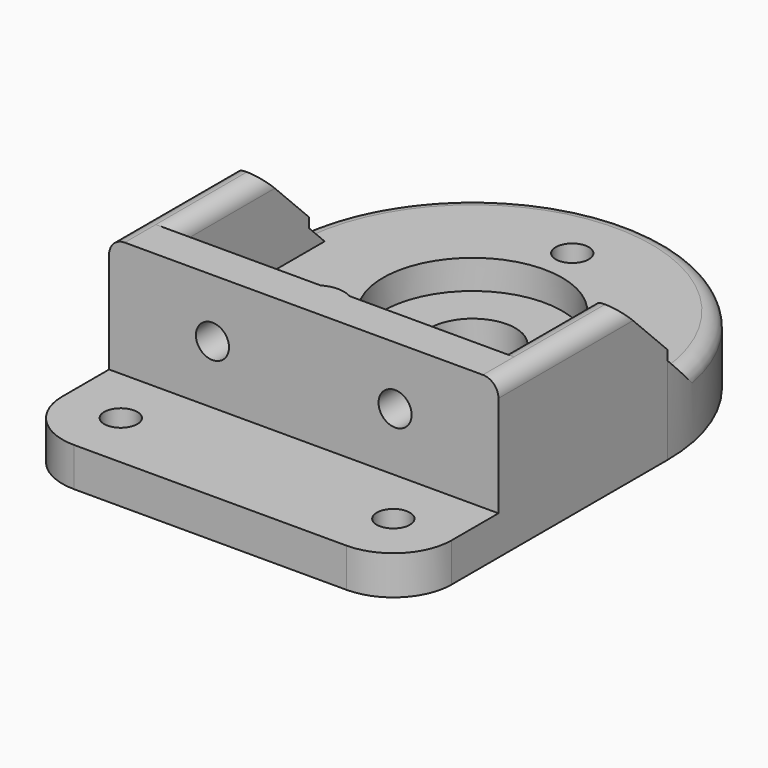
from build123d import *

# Parameters (mm, degrees)
F0_R          = 2.125
F0_R_2        = 5.25
F1_DEPTH      = 5
F3_DEPTH      = 15
F4_R          = 2.125
F5_DEPTH      = 25
F6_W          = 50
F6_H          = 15
F6_R          = 2.125
F7_DEPTH      = 5
F8_R          = 7.5
F9_SIZE       = 7.5
F10_R         = 2.125
F10_R_2       = 11.5
F11_DEPTH     = 3.75
F12_T1_DEPTH  = 10
F12_T6_DEPTH  = 4
F12_S7_R      = 25
F12_T8_DEPTH  = 4
F12_T12_DEPTH = 4
F12_S13_R     = 25
F12_T14_DEPTH = 4
F13_R         = 4.99999
F14_R         = 1.99999
F15_R         = 5.5
F16_DEPTH     = 25


# Not quite as in the source:
# - a fillet or chamfer that OpenCascade refuses, or shapes differently, is made with other operations: its cross-section is extruded or revolved along the edge and cut away or added
# - a fillet or chamfer is up to 0.001 mm smaller than in the source, because OpenCascade refuses the exact size


with BuildPart() as f1:
    # F0 (on Top) → F1 (new body)
    with BuildSketch(Plane.XY):
        with BuildLine():
            Line((25, -27.1), (25, -22.1))
            Line((25, -22.1), (25, 0))
            ThreePointArc((25, 0), (0, 25), (-25, 0))
            Line((-25, 0), (-25, -22.1))
            Line((-25, -22.1), (-25, -27.1))
            Line((-25, -27.1), (25, -27.1))
        make_face()
        with Locations((-13.8564064606, -8)):
            Circle(F0_R, mode=Mode.SUBTRACT)
        with Locations((13.8564064606, -8)):
            Circle(F0_R, mode=Mode.SUBTRACT)
        Circle(F0_R_2, mode=Mode.SUBTRACT)
        with Locations((0, 16)):
            Circle(F0_R, mode=Mode.SUBTRACT)
    extrude(amount=F1_DEPTH)

    # F2 (on face) → F3 (join)
    with BuildSketch(Plane.XY.offset(5)):
        Polygon((-25, -27.1), (25, -27.1), (25, -22.1), (25, 0), (21, 0), (21, -22.1), (5, -22.1), (5, -14.1), (0, -14.1), (-5, -14.1), (-5, -22.1), (-21, -22.1), (-21, 0), (-25, 0), (-25, -22.1), align=None)
    extrude(amount=F3_DEPTH)

    # F4 (on face) → F5 (cut)
    with BuildSketch(Plane.XZ.offset(27.1)):
        with Locations((-11.725, 12.5)):
            Circle(F4_R)
        with Locations((11.725, 12.5)):
            Circle(F4_R)
    extrude(amount=-F5_DEPTH, mode=Mode.SUBTRACT)

    # F6 (on Top) → F7 (join)
    with BuildSketch(Plane.XY):
        with Locations((0, -34.6)):
            Rectangle(F6_W, F6_H)
        with Locations((-17.5, -34.6)):
            Circle(F6_R, mode=Mode.SUBTRACT)
        with Locations((17.5, -34.6)):
            Circle(F6_R, mode=Mode.SUBTRACT)
    extrude(amount=F7_DEPTH)

    # F8
    f8_edges = [f1.edges().sort_by_distance(p)[0] for p in [
        (-25, -42.1, 2.5),
        (25, -42.1, 2.5),
    ]]
    fillet(f8_edges, radius=F8_R)

    # F9
    f9_edges = [f1.edges().sort_by_distance(p)[0] for p in [
        (0, -14.1, 20),
        (-23, 0, 20),
        (23, 0, 20),
    ]]
    chamfer(f9_edges, length=F9_SIZE)

    # F10 (on face) → F11 (join)
    with BuildSketch(Plane.XY.offset(5)):
        with BuildLine():
            Line((25, -22.1), (25, 0))
            ThreePointArc((25, 0), (0, 25), (-25, 0))
            Line((-25, 0), (-25, -22.1))
            Line((-25, -22.1), (25, -22.1))
        make_face()
        with Locations((-13.8564064606, -8)):
            Circle(F10_R, mode=Mode.SUBTRACT)
        Circle(F10_R_2, mode=Mode.SUBTRACT)
        with Locations((13.8564064606, -8)):
            Circle(F10_R, mode=Mode.SUBTRACT)
        with Locations((0, 16)):
            Circle(F10_R, mode=Mode.SUBTRACT)
    extrude(amount=F11_DEPTH)

    # F12: chamfer of 2.5 on 3 edges, made by hand

    # F12_s2 → F12_t1 (join)
    with BuildSketch(Plane.YZ.offset(-5)):
        with BuildLine():
            Line((-14.1707106781, 11.3207106781), (-11.5292893219, 8.6792893219))
            Line((-11.5292893219, 8.6792893219), (-11.5292893219, 8.6292893219))
            ThreePointArc((-11.5292893219, 8.6292893219), (-12.8146446609, 8.7), (-14.1, 8.7))
            Line((-14.1, 8.7), (-14.15, 8.75))
            ThreePointArc((-14.15, 8.75), (-14.15, 10.0353553391), (-14.2207106781, 11.3207106781))
            Line((-14.2207106781, 11.3207106781), (-14.1707106781, 11.3207106781))
        make_face()
    extrude(amount=F12_T1_DEPTH)


with BuildPart() as f12_tool4:
    # F12_s5 → F12_t6 (new body)
    with BuildSketch(Plane.YZ.offset(-21)):
        with BuildLine():
            Line((-0.0707106781, 11.3207106781), (2.5707106781, 8.6792893219))
            Line((2.5707106781, 8.6792893219), (2.5707106781, 8.6292893219))
            ThreePointArc((2.5707106781, 8.6292893219), (1.2853553391, 8.7), (0, 8.7))
            Line((0, 8.7), (-0.05, 8.75))
            ThreePointArc((-0.05, 8.75), (-0.05, 10.0353553391), (-0.1207106781, 11.3207106781))
            Line((-0.1207106781, 11.3207106781), (-0.0707106781, 11.3207106781))
        make_face()
    extrude(amount=-F12_T6_DEPTH)

    # F12_s7 → F12_t8 (intersect, symmetric)
    with BuildSketch(Plane.XY.offset(10)):
        Circle(F12_S7_R)
    extrude(amount=F12_T8_DEPTH, both=True, mode=Mode.INTERSECT)


with BuildPart() as f1_1:
    add(f1.part)

    # F12_t3: union F12_tool4
    add(f12_tool4.part)


with BuildPart() as f12_tool10:
    # F12_s11 → F12_t12 (new body)
    with BuildSketch(Plane.YZ.offset(25)):
        with BuildLine():
            Line((2.5707106781, 8.6792893219), (-0.0707106781, 11.3207106781))
            Line((-0.0707106781, 11.3207106781), (-0.1207106781, 11.3207106781))
            ThreePointArc((-0.1207106781, 11.3207106781), (-0.05, 10.0353553391), (-0.05, 8.75))
            Line((-0.05, 8.75), (0, 8.7))
            ThreePointArc((0, 8.7), (1.2853553391, 8.7), (2.5707106781, 8.6292893219))
            Line((2.5707106781, 8.6292893219), (2.5707106781, 8.6792893219))
        make_face()
    extrude(amount=-F12_T12_DEPTH)

    # F12_s13 → F12_t14 (intersect, symmetric)
    with BuildSketch(Plane.XY.offset(10)):
        Circle(F12_S13_R)
    extrude(amount=F12_T14_DEPTH, both=True, mode=Mode.INTERSECT)


with BuildPart() as f1_2:
    add(f1_1.part)

    # F12_t9: union F12_tool10
    add(f12_tool10.part)

    # F13 (radius 5 in the source; OpenCascade refuses exactly that, so slightly less here)
    f13_edges = [f1_2.edges().sort_by_distance(p)[0] for p in [
        (5, -17.85, 16.25),
        (-5, -17.85, 16.25),
    ]]
    fillet(f13_edges, radius=F13_R)

    # F14 (radius 2 in the source; OpenCascade refuses exactly that, so slightly less here)
    f14_edges = [f1_2.edges().sort_by_distance(p)[0] for p in [
        (21, -14.8, 20),
        (25, -17.3, 20),
        (-21, -14.8, 20),
        (-25, -17.3, 20),
        (0, 25, 8.75),
    ]]
    fillet(f14_edges, radius=F14_R)

    # F15 (on face) → F16 (cut)
    with BuildSketch(Plane.XY.offset(5)):
        Circle(F15_R)
    extrude(amount=-F16_DEPTH, mode=Mode.SUBTRACT)


solid = f1_2.part
